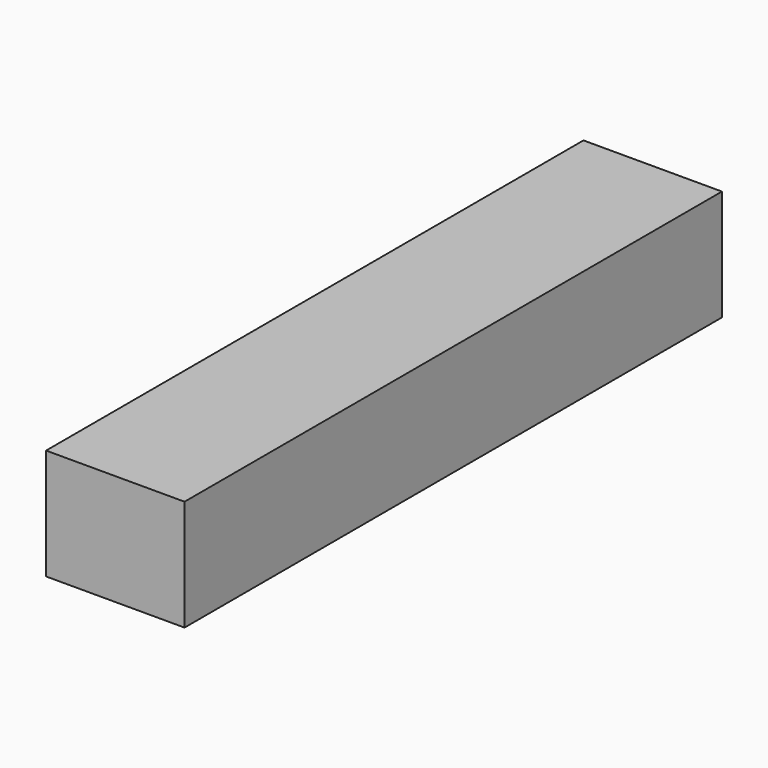
from build123d import *

# Parameters (mm, degrees)
F0_W     = 72.1459314227
F0_H     = 57.7507466078
F1_DEPTH = 350


# Not quite as in the source:
# - the program builds the solid bodies; features that only make, move or delete a surface that nothing else refers to are left out


with BuildPart() as f1:
    # F0 (on Front) → F1 (new body)
    with BuildSketch(Plane.XZ):
        with Locations((-36.0729657114, 28.8753733039)):
            Rectangle(F0_W, F0_H)
    extrude(amount=-F1_DEPTH)


solid = f1.part
